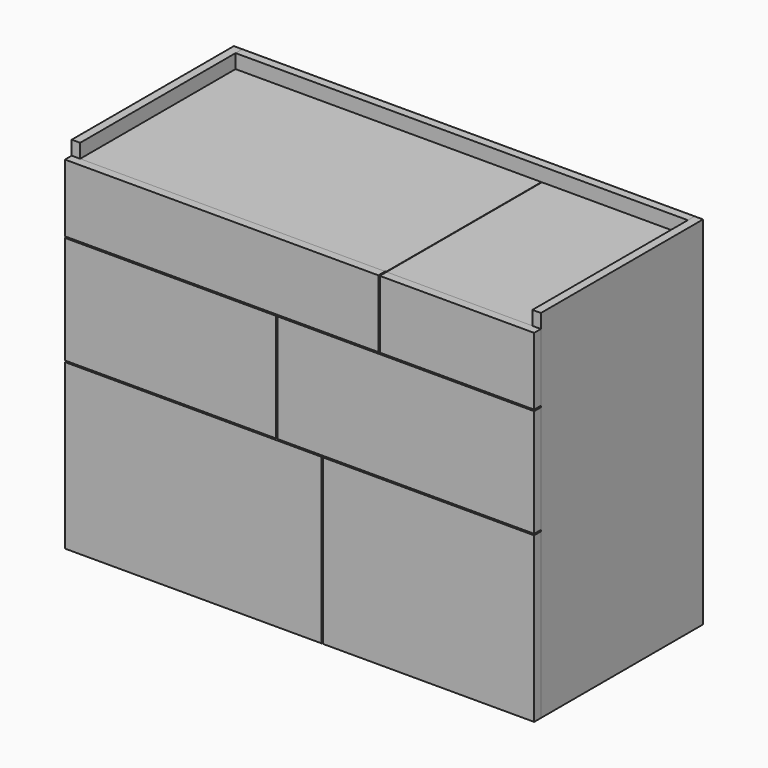
from build123d import *

# Parameters (mm, degrees)
F0_W           = 18
F0_H           = 414
F0_H_2         = 18
F1_DEPTH       = 760
F0_W_2         = 964
F2_DEPTH       = 760
F3_DEPTH       = 20
F3_DEPTH_BACK  = 10
F5_DEPTH       = 18
F4_W           = 652
F4_H           = 114
F4_H_2         = 300
F7_W           = 432
F7_H           = 230
F7_W_2         = 18
F8_DEPTH       = 18
F7_W_3         = 300
F7_W_4         = 244
F7_W_5         = 3
F7_W_6         = 450
F7_H_2         = 350
F7_W_7         = 226
F7_W_8         = 650
F7_H_3         = 80
F7_H_4         = 46
F7_H_5         = 18
F7_W_9         = 311
F10_DEPTH      = 414
F9_W           = 18
F9_H           = 9
F9_W_2         = 624.3935708242
F9_H_2         = 6
F9_H_3         = 3
F9_W_3         = 7.6064291758
F9_W_4         = 237.6064291758
F9_W_5         = 15
F9_W_6         = 10.3935708242
F9_H_4         = 15
F9_H_5         = 10
F11_DEPTH      = 414
F9_H_6         = 7.5
F9_H_7         = 170.74959
F9_H_8         = 291.25041
F9_H_9         = 120
F9_W_7         = 358.5
F12_DEPTH      = 400
F9_W_8         = 455.5
F9_H_10        = 190
F9_W_9         = 358.8239558978
F9_W_10        = 455.1760441022
F9_H_11        = 40
F9_H_12        = 87.5
F13_W          = 358.8239558978
F13_H          = 15
F13_W_2        = 15
F14_DEPTH      = 40
F14_DEPTH_BACK = 10
F13_W_3        = 485.1760441022
F16_W          = 642.3935708242
F16_H          = 12
F17_DEPTH      = 120
F19_DEPTH      = 18
F20_DEPTH      = 18


# Not quite as in the source:
# - a feature names something its author has since deleted; it is built from what else it names


with BuildPart() as f1:
    # F0 (on Top) → F1 (new body)
    with BuildSketch(Plane.XY):
        with Locations((9, 207)):
            Rectangle(F0_W, F0_H)
        with Locations((9, 423)):
            Rectangle(F0_W, F0_H_2)
    extrude(amount=F1_DEPTH)


with BuildPart() as f1b:
    # F0 (on Top) → F1, piece 2 (new body)
    with BuildSketch(Plane.XY):
        with Locations((991, 207)):
            Rectangle(F0_W, F0_H)
        with Locations((991, 423)):
            Rectangle(F0_W, F0_H_2)
    extrude(amount=F1_DEPTH)


with BuildPart() as f2:
    # F0 (on Top) → F2 (new body, through all)
    with BuildSketch(Plane.XY):
        with Locations((500, 423)):
            Rectangle(F0_W_2, F0_H_2)
    extrude(amount=F2_DEPTH)

    # F18 (on face) → F19 (cut, through all)
    with BuildSketch(Plane.XZ.offset(-414)):
        with BuildLine():
            ThreePointArc((60.5148148474, 607.3846153846), (65.5, 612), (70.4851851526, 607.3846153846))
            ThreePointArc((70.4851851526, 607.3846153846), (90.1806454277, 618.3548884782), (98, 639.5))
            ThreePointArc((98, 639.5), (44.3548884782, 664.1806454277), (60.5148148474, 607.3846153846))
        make_face()
        with BuildLine():
            ThreePointArc((59.0384615385, 609.6923076923), (65.5, 670), (71.9615384615, 609.6923076923))
            ThreePointArc((71.9615384615, 609.6923076923), (65.5, 614), (59.0384615385, 609.6923076923))
        make_face(mode=Mode.SUBTRACT)
        with BuildLine():
            ThreePointArc((60.5148148474, 607.3846153846), (65.5, 607), (70.4851851526, 607.3846153846))
            ThreePointArc((70.4851851526, 607.3846153846), (65.5, 612), (60.5148148474, 607.3846153846))
        make_face()
    extrude(amount=-F19_DEPTH, mode=Mode.SUBTRACT)


with BuildPart() as f3:
    # F0 (on Top) → F3 (new body, two sides)
    with BuildSketch(Plane.XY) as f3_sk:
        with Locations((500, 207)):
            Rectangle(F0_W_2, F0_H)
    extrude(amount=F3_DEPTH)
    extrude(f3_sk.sketch, amount=-F3_DEPTH_BACK)


with BuildPart() as f5:
    # F4 (on face) → F5 (new body)
    with BuildSketch(Plane.XY.offset(760)):
        Polygon((671, 0), (982, 0), (982, 414), (671, 414), (671, 300), align=None)
    extrude(amount=-F5_DEPTH)


with BuildPart() as f5b:
    # F4 (on face) → F5, piece 2 (new body)
    with BuildSketch(Plane.XY.offset(760)):
        with Locations((344, 357)):
            Rectangle(F4_W, F4_H)
        with Locations((344, 150)):
            Rectangle(F4_W, F4_H_2)
    extrude(amount=-F5_DEPTH)


with BuildPart() as f5_1:
    # F6: moved
    add(f5.part.moved(Location((0, 0, -30))))


with BuildPart() as f5b_1:
    # F6: moved
    add(f5b.part.moved(Location((0, 0, -30))))


with BuildPart() as f8:
    # F7 (on face) → F8 (new body)
    with BuildSketch(Plane.XZ):
        with Locations((234, 468)):
            Rectangle(F7_W, F7_H)
        with Locations((9, 468)):
            Rectangle(F7_W_2, F7_H)
    extrude(amount=F8_DEPTH)


with BuildPart() as f8b:
    # F7 (on face) → F8, piece 2 (new body)
    with BuildSketch(Plane.XZ):
        with Locations((603, 468)):
            Rectangle(F7_W_3, F7_H)
        with Locations((878, 468)):
            Rectangle(F7_W_4, F7_H)
        with Locations((754.5, 468)):
            Rectangle(F7_W_5, F7_H)
    extrude(amount=F8_DEPTH)


with BuildPart() as f8c:
    # F7 (on face) → F8, piece 3 (new body)
    with BuildSketch(Plane.XZ):
        with Locations((775, 175)):
            Rectangle(F7_W_6, F7_H_2)
    extrude(amount=F8_DEPTH)


with BuildPart() as f8d:
    # F7 (on face) → F8, piece 4 (new body)
    with BuildSketch(Plane.XZ):
        with Locations((397, 175)):
            Rectangle(F7_W_3, F7_H_2)
        with Locations((131, 175)):
            Rectangle(F7_W_7, F7_H_2)
        with Locations((9, 175)):
            Rectangle(F7_W_2, F7_H_2)
        with Locations((245.5, 175)):
            Rectangle(F7_W_5, F7_H_2)
    extrude(amount=F8_DEPTH)


with BuildPart() as f8e:
    # F7 (on face) → F8, piece 5 (new body)
    with BuildSketch(Plane.XZ):
        with Locations((343, 626)):
            Rectangle(F7_W_8, F7_H_3)
        with Locations((9, 626)):
            Rectangle(F7_W_2, F7_H_3)
        with Locations((9, 689)):
            Rectangle(F7_W_2, F7_H_4)
        with Locations((343, 689)):
            Rectangle(F7_W_8, F7_H_4)
        with Locations((343, 721)):
            Rectangle(F7_W_8, F7_H_5)
        with Locations((9, 721)):
            Rectangle(F7_W_2, F7_H_5)
    extrude(amount=F8_DEPTH)


with BuildPart() as f8f:
    # F7 (on face) → F8, piece 6 (new body)
    with BuildSketch(Plane.XZ):
        Polygon((1000, 730), (671, 730), (671, 604), (982, 604), (982, 586), (1000, 586), align=None)
        with Locations((826.5, 595)):
            Rectangle(F7_W_9, F7_H_5)
    extrude(amount=F8_DEPTH)


with BuildPart() as f10:
    # F9 (on face) → F10 (new body, through all)
    with BuildSketch(Plane(origin=(0, 0, 0), x_dir=(-1, 0, 0), z_dir=(0, 1, 0))):
        Polygon((-18, 361.75041), (-36, 361.75041), (-51, 361.75041), (-442.5, 361.75041), (-460.5, 361.75041), (-964, 361.75041), (-982, 361.75041), (-982, 343.75041), (-964, 343.75041), (-949, 343.75041), (-590.1760441022, 343.75041), (-575.1760441022, 343.75041), (-557.1760441022, 343.75041), (-539.1760441022, 343.75041), (-521.1760441022, 343.75041), (-506.1760441022, 343.75041), (-51, 343.75041), (-36, 343.75041), (-18, 343.75041), align=None)
    extrude(amount=F10_DEPTH)


with BuildPart() as f10b:
    # F9 (on face) → F10, piece 2 (new body, through all)
    with BuildSketch(Plane(origin=(0, 0, 0), x_dir=(-1, 0, 0), z_dir=(0, 1, 0))):
        Polygon((-18, 574), (-18, 583), (-36, 583), (-660.3935708242, 583), (-678.3935708242, 583), (-696.3935708242, 583), (-711.3935708242, 583), (-949, 583), (-964, 583), (-982, 583), (-982, 574), (-424.5, 574), (-409.5, 574), align=None)
        with Locations((-687.3935708242, 587.5)):
            Rectangle(F9_W, F9_H)
        Polygon((-678.3935708242, 583), (-660.3935708242, 583), (-660.3935708242, 586), (-668, 586), (-668, 592), (-678.3935708242, 592), align=None)
        with Locations((-973, 587.5)):
            Rectangle(F9_W, F9_H)
        with Locations((-348.1967854121, 589)):
            Rectangle(F9_W_2, F9_H_2)
        with Locations((-27, 589)):
            Rectangle(F9_W, F9_H_2)
        with Locations((-27, 584.5)):
            Rectangle(F9_W, F9_H_3)
        with Locations((-348.1967854121, 584.5)):
            Rectangle(F9_W_2, F9_H_3)
        with Locations((-664.1967854121, 589)):
            Rectangle(F9_W_3, F9_H_2)
        with Locations((-830.1967854121, 587.5)):
            Rectangle(F9_W_4, F9_H)
        with Locations((-956.5, 587.5)):
            Rectangle(F9_W_5, F9_H)
        with Locations((-703.8935708242, 587.5)):
            Rectangle(F9_W_5, F9_H)
    extrude(amount=F10_DEPTH)


with BuildPart() as f11:
    # F9 (on face) → F11 (new body, through all)
    with BuildSketch(Plane(origin=(0, 0, 0), x_dir=(-1, 0, 0), z_dir=(0, 1, 0))):
        Polygon((-668, 617), (-668, 712), (-678.3935708242, 712), (-678.3935708242, 704.5), (-678.3935708242, 617), align=None)
        Polygon((-668, 592), (-660.3935708242, 592), (-660.3935708242, 712), (-668, 712), (-668, 617), (-668, 607), align=None)
        with Locations((-673.1967854121, 599.5)):
            Rectangle(F9_W_6, F9_H_4)
        with Locations((-673.1967854121, 612)):
            Rectangle(F9_W_6, F9_H_5)
    extrude(amount=F11_DEPTH)


with BuildPart() as f11b:
    # F9 (on face) → F11, piece 2 (new body, through all)
    with BuildSketch(Plane(origin=(0, 0, 0), x_dir=(-1, 0, 0), z_dir=(0, 1, 0))):
        with Locations((-451.5, 561.25)):
            Rectangle(F9_W, F9_H_6)
        with Locations((-451.5, 472.125205)):
            Rectangle(F9_W, F9_H_7)
        with Locations((-451.5, 381.75041)):
            Rectangle(F9_W, F9_H_5)
        with Locations((-451.5, 369.25041)):
            Rectangle(F9_W, F9_H_4)
    extrude(amount=F11_DEPTH)


with BuildPart() as f11c:
    # F9 (on face) → F11, piece 3 (new body, through all)
    with BuildSketch(Plane(origin=(0, 0, 0), x_dir=(-1, 0, 0), z_dir=(0, 1, 0))):
        with Locations((-548.1760441022, 340.00041)):
            Rectangle(F9_W, F9_H_6)
        with Locations((-548.1760441022, 190.625205)):
            Rectangle(F9_W, F9_H_8)
        with Locations((-548.1760441022, 40)):
            Rectangle(F9_W, F9_H_5)
        with Locations((-548.1760441022, 27.5)):
            Rectangle(F9_W, F9_H_4)
    extrude(amount=F11_DEPTH)


with BuildPart() as f11d:
    # F9 (on face) → F11, piece 4 (new body, through all)
    with BuildSketch(Plane(origin=(0, 0, 0), x_dir=(-1, 0, 0), z_dir=(0, 1, 0))):
        with Locations((-973, 708.25)):
            Rectangle(F9_W, F9_H_6)
    extrude(amount=F11_DEPTH)


with BuildPart() as f11e:
    # F9 (on face) → F11, piece 5 (new body, through all)
    with BuildSketch(Plane(origin=(0, 0, 0), x_dir=(-1, 0, 0), z_dir=(0, 1, 0))):
        with Locations((-27, 652)):
            Rectangle(F9_W, F9_H_9)
    extrude(amount=F11_DEPTH)


with BuildPart() as f12:
    # F9 (on face) → F12 (new body)
    with BuildSketch(Plane(origin=(0, 0, 0), x_dir=(-1, 0, 0), z_dir=(0, 1, 0))):
        with Locations((-43.5, 472.125205)):
            Rectangle(F9_W_5, F9_H_7)
        with Locations((-43.5, 381.75041)):
            Rectangle(F9_W_5, F9_H_5)
        with Locations((-230.25, 381.75041)):
            Rectangle(F9_W_7, F9_H_5)
        with Locations((-417, 381.75041)):
            Rectangle(F9_W_5, F9_H_5)
        with Locations((-417, 472.125205)):
            Rectangle(F9_W_5, F9_H_7)
    extrude(amount=F12_DEPTH)


with BuildPart() as f12b:
    # F9 (on face) → F12, piece 2 (new body)
    with BuildSketch(Plane(origin=(0, 0, 0), x_dir=(-1, 0, 0), z_dir=(0, 1, 0))):
        with Locations((-486, 472.125205)):
            Rectangle(F9_W_5, F9_H_7)
        with Locations((-486, 381.75041)):
            Rectangle(F9_W_5, F9_H_5)
        with Locations((-721.25, 381.75041)):
            Rectangle(F9_W_8, F9_H_5)
        with Locations((-956.5, 381.75041)):
            Rectangle(F9_W_5, F9_H_5)
        with Locations((-956.5, 472.125205)):
            Rectangle(F9_W_5, F9_H_7)
    extrude(amount=F12_DEPTH)


with BuildPart() as f12c:
    # F9 (on face) → F12, piece 3 (new body)
    with BuildSketch(Plane(origin=(0, 0, 0), x_dir=(-1, 0, 0), z_dir=(0, 1, 0))):
        with Locations((-956.5, 140)):
            Rectangle(F9_W_5, F9_H_10)
        with Locations((-956.5, 40)):
            Rectangle(F9_W_5, F9_H_5)
        with Locations((-769.5880220511, 40)):
            Rectangle(F9_W_9, F9_H_5)
        with Locations((-582.6760441022, 40)):
            Rectangle(F9_W_5, F9_H_5)
        with Locations((-582.6760441022, 140)):
            Rectangle(F9_W_5, F9_H_10)
    extrude(amount=F12_DEPTH)


with BuildPart() as f12d:
    # F9 (on face) → F12, piece 4 (new body)
    with BuildSketch(Plane(origin=(0, 0, 0), x_dir=(-1, 0, 0), z_dir=(0, 1, 0))):
        with Locations((-513.6760441022, 40)):
            Rectangle(F9_W_5, F9_H_5)
        with Locations((-513.6760441022, 140)):
            Rectangle(F9_W_5, F9_H_10)
        with Locations((-278.5880220511, 40)):
            Rectangle(F9_W_10, F9_H_5)
        with Locations((-43.5, 40)):
            Rectangle(F9_W_5, F9_H_5)
        with Locations((-43.5, 140)):
            Rectangle(F9_W_5, F9_H_10)
    extrude(amount=F12_DEPTH)


with BuildPart() as f12e:
    # F9 (on face) → F12, piece 5 (new body)
    with BuildSketch(Plane(origin=(0, 0, 0), x_dir=(-1, 0, 0), z_dir=(0, 1, 0))):
        with Locations((-513.6760441022, 283.75041)):
            Rectangle(F9_W_5, F9_H_11)
        with Locations((-513.6760441022, 258.75041)):
            Rectangle(F9_W_5, F9_H_5)
        with Locations((-278.5880220511, 258.75041)):
            Rectangle(F9_W_10, F9_H_5)
        with Locations((-43.5, 258.75041)):
            Rectangle(F9_W_5, F9_H_5)
        with Locations((-43.5, 283.75041)):
            Rectangle(F9_W_5, F9_H_11)
    extrude(amount=F12_DEPTH)


with BuildPart() as f12f:
    # F9 (on face) → F12, piece 6 (new body)
    with BuildSketch(Plane(origin=(0, 0, 0), x_dir=(-1, 0, 0), z_dir=(0, 1, 0))):
        with Locations((-582.6760441022, 283.75041)):
            Rectangle(F9_W_5, F9_H_11)
        with Locations((-582.6760441022, 258.75041)):
            Rectangle(F9_W_5, F9_H_5)
        with Locations((-769.5880220511, 258.75041)):
            Rectangle(F9_W_9, F9_H_5)
        with Locations((-956.5, 283.75041)):
            Rectangle(F9_W_5, F9_H_11)
        with Locations((-956.5, 258.75041)):
            Rectangle(F9_W_5, F9_H_5)
    extrude(amount=F12_DEPTH)


with BuildPart() as f12g:
    # F9 (on face) → F12, piece 7 (new body)
    with BuildSketch(Plane(origin=(0, 0, 0), x_dir=(-1, 0, 0), z_dir=(0, 1, 0))):
        with Locations((-956.5, 660.75)):
            Rectangle(F9_W_5, F9_H_12)
        with Locations((-703.8935708242, 660.75)):
            Rectangle(F9_W_5, F9_H_12)
        with Locations((-703.8935708242, 612)):
            Rectangle(F9_W_5, F9_H_5)
        with Locations((-830.1967854121, 612)):
            Rectangle(F9_W_4, F9_H_5)
        with Locations((-956.5, 612)):
            Rectangle(F9_W_5, F9_H_5)
    extrude(amount=F12_DEPTH)


with BuildPart() as f14:
    # F13 (on face) → F14 (new body, two sides)
    with BuildSketch(Plane.XY.offset(263.75041)) as f14_sk:
        with Locations((769.5880220511, 7.5)):
            Rectangle(F13_W, F13_H)
        with Locations((956.5, 7.5)):
            Rectangle(F13_W_2, F13_H)
        with Locations((582.6760441022, 7.5)):
            Rectangle(F13_W_2, F13_H)
    extrude(amount=F14_DEPTH)
    extrude(f14_sk.sketch, amount=-F14_DEPTH_BACK)


with BuildPart() as f14b:
    # F13 (on face) → F14, piece 2 (new body, two sides)
    with BuildSketch(Plane.XY.offset(263.75041)) as f14_2_sk:
        with Locations((278.5880220511, 7.5)):
            Rectangle(F13_W_3, F13_H)
    extrude(amount=F14_DEPTH)
    extrude(f14_2_sk.sketch, amount=-F14_DEPTH_BACK)


with BuildPart() as f12f_1:
    add(f12f.part)

    # F15: cut F14, F14b
    add(f14.part, mode=Mode.SUBTRACT)
    add(f14b.part, mode=Mode.SUBTRACT)


with BuildPart() as f12e_1:
    add(f12e.part)

    # F15: cut F14, F14b
    add(f14.part, mode=Mode.SUBTRACT)
    add(f14b.part, mode=Mode.SUBTRACT)


with BuildPart() as f17:
    # F16 (on face) → F17 (new body, through all)
    with BuildSketch(Plane.XY.offset(592)):
        with Locations((339.1967854121, 6)):
            Rectangle(F16_W, F16_H)
    extrude(amount=F17_DEPTH)


with BuildPart() as f20:
    # F18 (on face) → F20 (new body, through all)
    with BuildSketch(Plane.XZ.offset(-414)):
        with BuildLine():
            ThreePointArc((60.5148148474, 607.3846153846), (65.5, 612), (70.4851851526, 607.3846153846))
            ThreePointArc((70.4851851526, 607.3846153846), (90.1806454277, 618.3548884782), (98, 639.5))
            ThreePointArc((98, 639.5), (44.3548884782, 664.1806454277), (60.5148148474, 607.3846153846))
        make_face()
        with BuildLine():
            ThreePointArc((59.0384615385, 609.6923076923), (65.5, 670), (71.9615384615, 609.6923076923))
            ThreePointArc((71.9615384615, 609.6923076923), (65.5, 614), (59.0384615385, 609.6923076923))
        make_face(mode=Mode.SUBTRACT)
    extrude(amount=-F20_DEPTH)


solid = Compound([f1.part, f1b.part, f2.part, f3.part, f5_1.part, f5b_1.part, f8.part, f8b.part, f8c.part, f8d.part, f8e.part, f8f.part, f10.part, f10b.part, f11.part, f11b.part, f11c.part, f11d.part, f11e.part, f12.part, f12b.part, f12c.part, f12d.part, f12g.part, f14.part, f14b.part, f12f_1.part, f12e_1.part, f17.part, f20.part])
